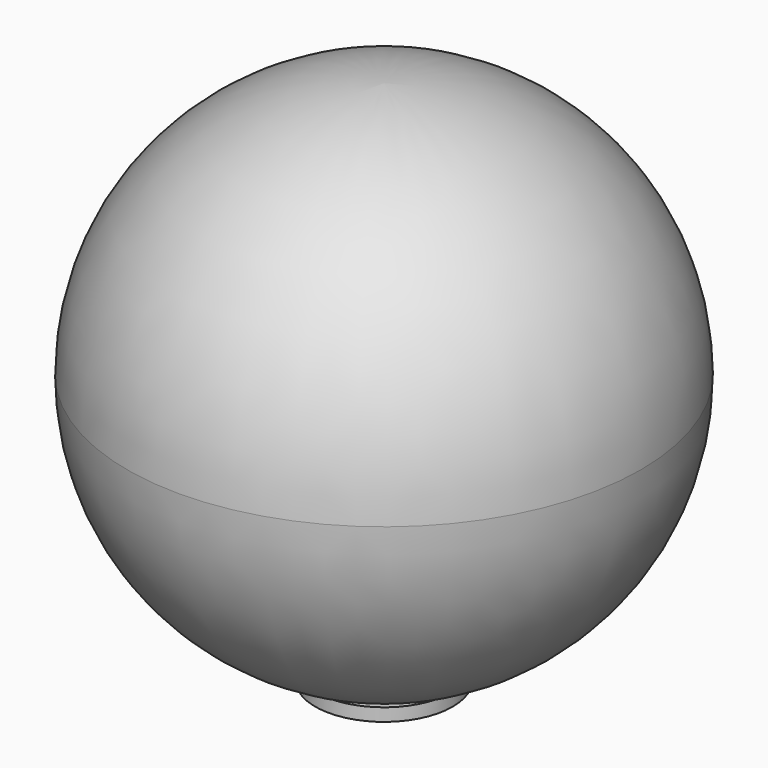
from build123d import *

# Parameters (mm, degrees)
F0_R     = 40
F1_DEPTH = 80
F2_R     = 39.99999
F3_R     = 10.7068086525
F4_DEPTH = 2


# Not quite as in the source:
# - a fillet or chamfer is up to 0.001 mm smaller than in the source, because OpenCascade refuses the exact size


with BuildPart() as f1:
    # F0 (on Top) → F1 (new body)
    with BuildSketch(Plane.XY):
        Circle(F0_R)
    extrude(amount=F1_DEPTH)

    # F2 (radius 40 in the source; OpenCascade refuses exactly that, so slightly less here)
    f2_edges = [f1.edges().sort_by_distance(p)[0] for p in [
        (-40, 0, 80),
        (-40, 0, 0),
    ]]
    fillet(f2_edges, radius=F2_R)


with BuildPart() as f4:
    # F3 (on Top) → F4 (new body)
    with BuildSketch(Plane.XY):
        Circle(F3_R)
    extrude(amount=-F4_DEPTH)


solid = Compound([f1.part, f4.part])
